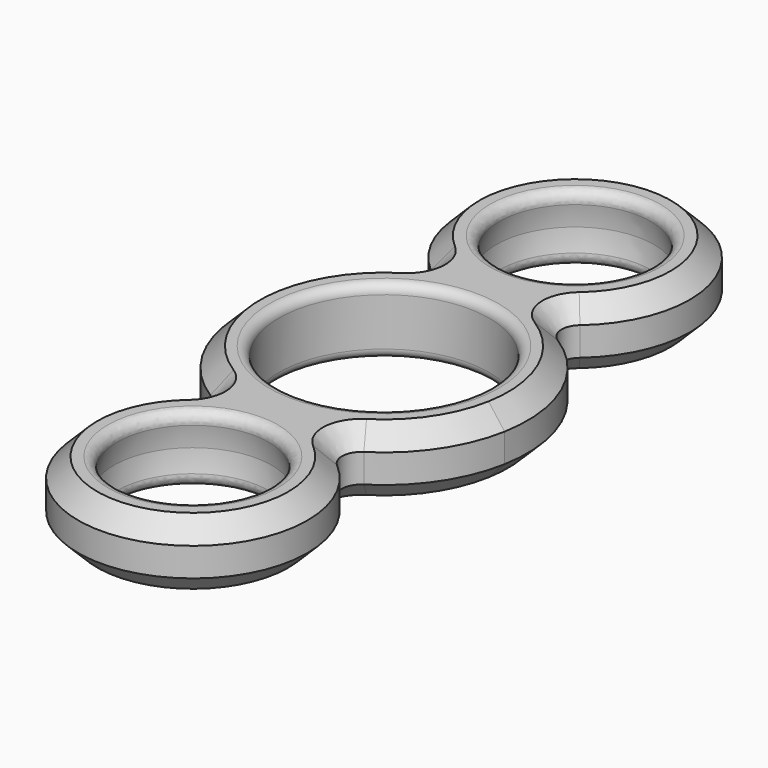
from build123d import *

# Parameters (mm, degrees)
F0_R     = 8.25
F0_R_2   = 11
F1_DEPTH = 7
F2_R     = 2
F3_SIZE  = 2
F9_R     = 1


# Not quite as in the source:
# - a pattern or mirror of a feature is missing from the dataset's text; its kind, count and spacing are read off the source's solid
# - a feature names something its author has since deleted; it is built from what else it names


with BuildPart() as f1:
    # F0 (on Top) → F1 (new body)
    with BuildSketch(Plane.XY):
        with BuildLine():
            ThreePointArc((14.7593654246, -2.6760291972), (12.9903810568, 7.5), (5.0621734463, 14.12))
            ThreePointArc((5.0621734463, 14.12), (0, 37), (-5.0621734463, 14.12))
            ThreePointArc((-5.0621734463, 14.12), (-15, 0), (-5.0621734463, -14.12))
            ThreePointArc((-5.0621734463, -14.12), (0, -37), (5.0621734463, -14.12))
            ThreePointArc((5.0621734463, -14.12), (11.4439708028, -9.6971919783), (14.7593654246, -2.6760291972))
        make_face()
        with Locations((0, -25)):
            Circle(F0_R, mode=Mode.SUBTRACT)
        Circle(F0_R_2, mode=Mode.SUBTRACT)
        with Locations((0, 25)):
            Circle(F0_R, mode=Mode.SUBTRACT)
    extrude(amount=F1_DEPTH)

    # F2
    f2_edges = [f1.edges().sort_by_distance(p)[0] for p in [
        (5.062173, -14.12, 3.5),
        (5.062173, 14.12, 3.5),
        (-5.062173, 14.12, 3.5),
        (-5.062173, -14.12, 3.5),
    ]]
    fillet(f2_edges, radius=F2_R)

    # F3
    f3_edges = [f1.edges().sort_by_distance(p)[0] for p in [
        (0, -37, 7),
        (0, -37, 0),
        (15, 0, 7),
        (15, 0, 0),
        (7.104012, 14.217419, 7),
        (7.104012, -14.217419, 7),
        (0, 37, 7),
        (-7.104012, 14.217419, 7),
        (-7.104012, -14.217419, 7),
        (-15, 0, 7),
        (7.104012, 14.217419, 0),
        (7.104012, -14.217419, 0),
        (0, 37, 0),
        (-7.104012, -14.217419, 0),
        (-7.104012, 14.217419, 0),
        (-15, 0, 0),
    ]]
    chamfer(f3_edges, length=F3_SIZE)

    # F7 (on 3pt) → F8 (revolve)
    with BuildSketch(Plane.YZ):
        with BuildLine():
            Line((-32.4707763987, 7), (-33.25, 7))
            Line((-33.25, 7), (-33.25, 3.5))
            ThreePointArc((-33.25, 3.5), (-33.0528381733, 5.2928461605), (-32.4707763987, 7))
        make_face()
        with BuildLine():
            ThreePointArc((-32.4707763987, 0), (-33.0528381733, 1.7071538395), (-33.25, 3.5))
            Line((-33.25, 3.5), (-33.25, 0))
            Line((-33.25, 0), (-32.4707763987, 0))
        make_face()
    f8 = revolve(axis=Axis((0, -25, 3.5), (0, 0, 1)))

    # F8_copies: F8 across plane
    add(f8.mirror(Plane.ZX))

    # F9
    f9_edges = [f1.edges().sort_by_distance(p)[0] for p in [
        (0, -17.529224, 7),
        (0, -17.529224, 0),
        (-11, 0, 0),
        (-11, 0, 7),
        (0, 17.529224, 7),
        (0, 17.529224, 0),
    ]]
    fillet(f9_edges, radius=F9_R)


solid = f1.part
